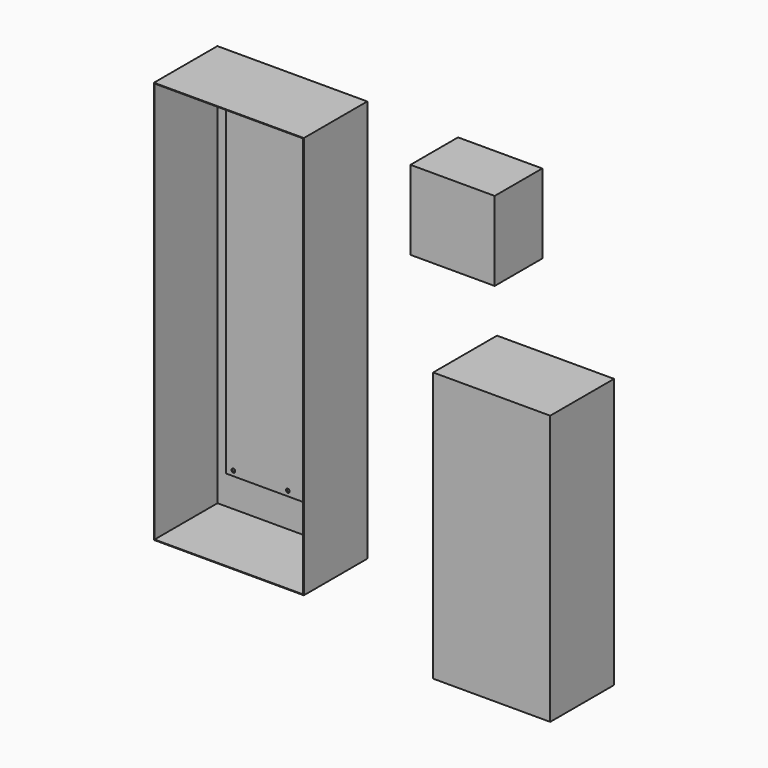
from build123d import *

# Parameters (mm, degrees)
F0_W     = 762
F0_H     = 3.175
F0_H_2   = 2057.4
F1_DEPTH = 3.175
F2_DEPTH = 406.4
F4_START = 19.05
F3_W     = 635
F3_H     = 101.6
F3_R     = 9.525
F3_H_2   = 1562.1
F3_H_3   = 63.5
F4_DEPTH = 6.35
F3_W_2   = 431.8
F3_H_4   = 406.4
F5_DEPTH = 304.8
F3_W_3   = 600
F3_H_5   = 1382
F6_DEPTH = 409


# Not quite as in the source:
# - a length typed as a fraction of an inch, garbled in the dataset ("3 / 203.2 mm" for 3/8 in), is restored


with BuildPart() as f1:
    # F0 (on Front) → F1 (new body)
    with BuildSketch(Plane.XZ):
        Polygon((381, -1028.7), (-381, -1028.7), (-384.175, -1028.7), (-384.175, -1031.875), (384.175, -1031.875), (384.175, -1028.7), align=None)
        Polygon((-381, -1028.7), (-381, 1028.7), (-381, 1031.875), (-384.175, 1031.875), (-384.175, -1028.7), align=None)
        Polygon((381, 1031.875), (381, 1028.7), (381, -1028.7), (384.175, -1028.7), (384.175, 1031.875), align=None)
        with Locations((0, 1030.2875)):
            Rectangle(F0_W, F0_H)
        Rectangle(F0_W, F0_H_2)
    extrude(amount=F1_DEPTH)

    # F0 (on Front) → F2 (join)
    with BuildSketch(Plane.XZ):
        Polygon((-381, -1028.7), (-381, 1028.7), (-381, 1031.875), (-384.175, 1031.875), (-384.175, -1028.7), align=None)
        with Locations((0, 1030.2875)):
            Rectangle(F0_W, F0_H)
        Polygon((381, 1031.875), (381, 1028.7), (381, -1028.7), (384.175, -1028.7), (384.175, 1031.875), align=None)
        Polygon((381, -1028.7), (-381, -1028.7), (-384.175, -1028.7), (-384.175, -1031.875), (384.175, -1031.875), (384.175, -1028.7), align=None)
    extrude(amount=F2_DEPTH)


with BuildPart() as f4:
    # F3 (on face) → F4 (new body)
    with BuildSketch(Plane.XZ.offset(3.175).offset(F4_START)):
        with Locations((0, 812.8)):
            Rectangle(F3_W, F3_H)
        with Locations((-279.4, 838.2)):
            Circle(F3_R, mode=Mode.SUBTRACT)
        with Locations((0, 838.2)):
            Circle(F3_R, mode=Mode.SUBTRACT)
        with Locations((279.4, 838.2)):
            Circle(F3_R, mode=Mode.SUBTRACT)
        with Locations((0, -19.05)):
            Rectangle(F3_W, F3_H_2)
        with Locations((0, -831.85)):
            Rectangle(F3_W, F3_H_3)
        with Locations((-279.4, -838.2)):
            Circle(F3_R, mode=Mode.SUBTRACT)
        with Locations((0, -838.2)):
            Circle(F3_R, mode=Mode.SUBTRACT)
        with Locations((279.4, -838.2)):
            Circle(F3_R, mode=Mode.SUBTRACT)
    extrude(amount=F4_DEPTH)


with BuildPart() as f5:
    # F3 (on face) → F5 (new body)
    with BuildSketch(Plane.XZ.offset(3.175)):
        with Locations((1067.8818782806, 820.0628931046)):
            Rectangle(F3_W_2, F3_H_4)
    extrude(amount=F5_DEPTH)


with BuildPart() as f6:
    # F3 (on face) → F6 (new body)
    with BuildSketch(Plane.XZ.offset(3.175)):
        with Locations((1351.792383194, -497.5234422684)):
            Rectangle(F3_W_3, F3_H_5)
    extrude(amount=F6_DEPTH)


solid = Compound([f1.part, f4.part, f5.part, f6.part])
